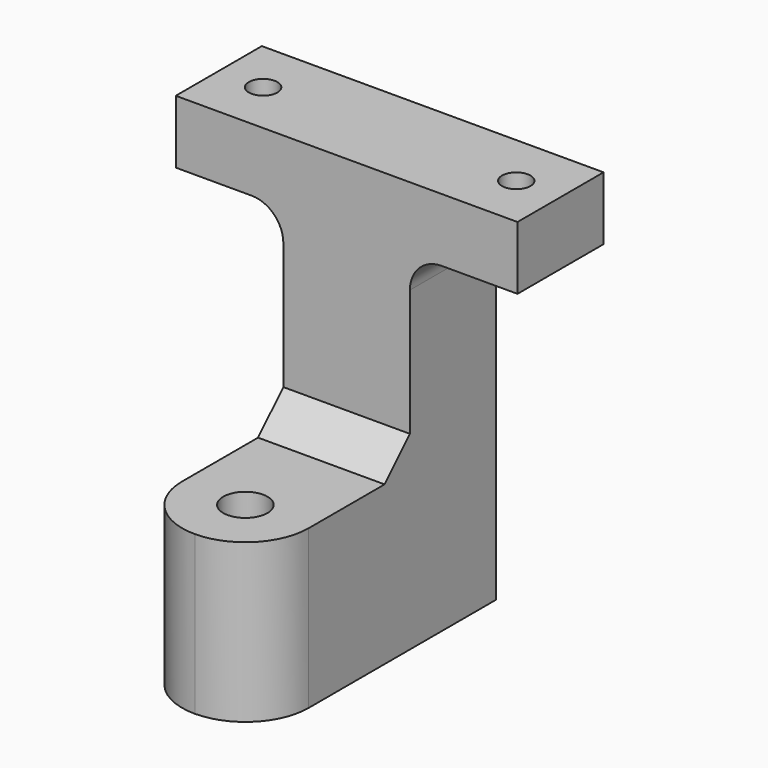
from build123d import *

# Parameters (mm, degrees)
F1_DEPTH = 47
F3_D     = 7
F4_W     = 54
F4_H     = 30
F5_DEPTH = 40.001
F6_R     = 9.99999
F8_R     = 5
F10_D    = 4.5
F11_SIZE = 5


# Not quite as in the source:
# - a fillet or chamfer is up to 0.001 mm smaller than in the source, because OpenCascade refuses the exact size


with BuildPart() as f1:
    # F0 (on Front) → F1 (new body)
    with BuildSketch(Plane.XZ):
        Polygon((27, 40), (-27, 40), (-27, 30), (-10, 30), (-10, -25), (10, -25), (10, 30), (27, 30), align=None)
    extrude(amount=F1_DEPTH)

    # F3 (through all)
    with Locations(Plane(origin=(0, 0, -25), x_dir=(1, 0, 0), z_dir=(0, 0, -1))):
        with Locations((0, 37)):
            Hole(F3_D / 2)

    # F4 (on Top) → F5 (cut, through all)
    with BuildSketch(Plane.XY):
        with Locations((0, -32)):
            Rectangle(F4_W, F4_H)
    extrude(amount=F5_DEPTH, mode=Mode.SUBTRACT)

    # F6 (radius 10 in the source; OpenCascade refuses exactly that, so slightly less here)
    f6_edges = [f1.edges().sort_by_distance(p)[0] for p in [
        (-10, -47, -12.5),
        (10, -47, -12.5),
    ]]
    fillet(f6_edges, radius=F6_R)

    # F8
    f8_edges = [f1.edges().sort_by_distance(p)[0] for p in [
        (10, -8.5, 30),
        (-10, -8.5, 30),
    ]]
    fillet(f8_edges, radius=F8_R)

    # F10 (through all)
    with Locations(Plane.XY.offset(40)):
        with Locations((-20, -8.5), (20, -8.5)):
            Hole(F10_D / 2)

    # F11
    f11_edges = [f1.edges().sort_by_distance(p)[0] for p in [
        (0, -17, 0),
    ]]
    chamfer(f11_edges, length=F11_SIZE)


solid = f1.part
